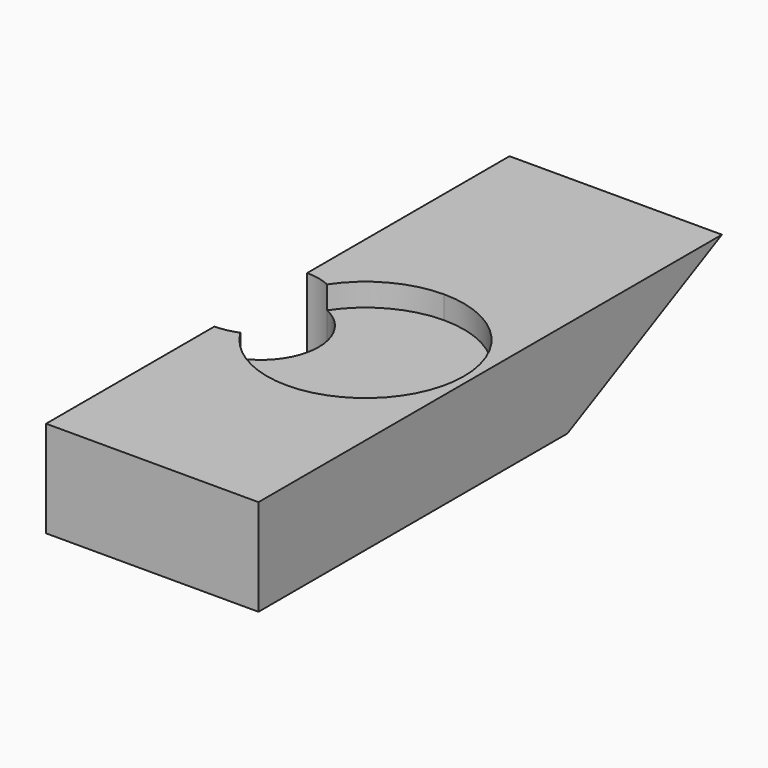
from build123d import *

# Parameters (mm, degrees)
F1_DEPTH = 27.94
F3_DEPTH = 3
F5_DEPTH = 25.4


with BuildPart() as f1:
    # F0 (on Right) → F1 (new body)
    with BuildSketch(Plane.YZ):
        Polygon((0, 12.7), (0, 0), (50.8, 0), (76.2, 12.7), align=None)
    extrude(amount=F1_DEPTH)

    # F2 (on face) → F3 (cut)
    with BuildSketch(Plane.XY.offset(12.7)):
        with BuildLine():
            ThreePointArc((13.97, 48.006), (1.016, 35.052), (13.97, 22.098))
            Line((13.97, 22.098), (13.97, 48.006))
        make_face()
        with BuildLine():
            Line((13.97, 48.006), (13.97, 22.098))
            ThreePointArc((13.97, 22.098), (23.1298612435, 25.8921387565), (26.924, 35.052))
            ThreePointArc((26.924, 35.052), (23.1298612435, 44.2118612435), (13.97, 48.006))
        make_face()
    extrude(amount=-F3_DEPTH, mode=Mode.SUBTRACT)

    # F4 (on face) → F5 (cut)
    with BuildSketch(Plane.XY.offset(12.7)):
        with BuildLine():
            ThreePointArc((2.9316641234, 28.2725267849), (1.0181406263, 35.2874883522), (3.1854046142, 42.2282537835))
            ThreePointArc((3.1854046142, 42.2282537835), (1.6304640704, 42.7495197934), (0, 42.926))
            Line((0, 42.926), (0, 27.686))
            ThreePointArc((0, 27.686), (1.4948802796, 27.8340703329), (2.9316641234, 28.2725267849))
        make_face()
        with BuildLine():
            ThreePointArc((2.9316641234, 28.2725267849), (6.3404921189, 31.0795878466), (7.62, 35.306))
            ThreePointArc((7.62, 35.306), (6.4162755225, 39.4164511212), (3.1854046142, 42.2282537835))
            ThreePointArc((3.1854046142, 42.2282537835), (1.0181406263, 35.2874883522), (2.9316641234, 28.2725267849))
        make_face()
    extrude(amount=-F5_DEPTH, mode=Mode.SUBTRACT)


solid = f1.part
